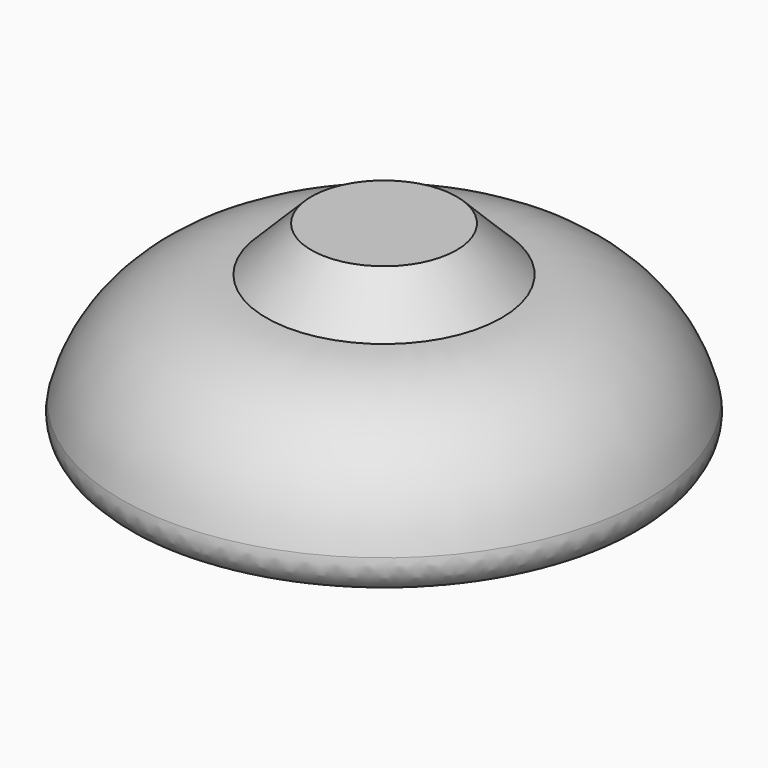
from build123d import *

# Parameters (mm, degrees)
F0_R     = 45.3065751062
F1_DEPTH = 25.4
F2_R     = 25.39999
F3_R     = 5.08
F4_T     = 2.54
F5_DEPTH = 7.62
F6_SIZE  = 7.61999
F7_DEPTH = 20.32
F8_R     = 19.812


# Not quite as in the source:
# - a fillet or chamfer is up to 0.001 mm smaller than in the source, because OpenCascade refuses the exact size
# - a shell that OpenCascade refuses in one call is made with other operations: the cavity is built on its own and cut out


with BuildPart() as f1:
    # F0 (on Top) → F1 (new body)
    with BuildSketch(Plane.XY):
        Circle(F0_R)
    extrude(amount=F1_DEPTH)

    # F2 (radius 25.4 in the source; OpenCascade refuses exactly that, so slightly less here)
    f2_edges = [f1.edges().sort_by_distance(p)[0] for p in [
        (-45.306575, 0, 25.4),
    ]]
    fillet(f2_edges, radius=F2_R)

    # F3
    f3_edges = [f1.edges().sort_by_distance(p)[0] for p in [
        (-45.306575, 0, 0),
    ]]
    fillet(f3_edges, radius=F3_R)

    # F4: shell of thickness 2.54, made by hand


with BuildPart() as f4_core1:
    # F4_t2: copy of F1
    add(f1.part)

    # the walls: a layer under each face that stays
    f4_faces = [f4_core1.faces().sort_by_distance(p)[0] for p in [
        (-35.4608426764, 0, 20.0804622717),
        (-43.5974247944, 0, 1.9691472612),
        (0, 0, 25.4),
    ]]
    thicken(f4_faces, amount=-F4_T, mode=Mode.SUBTRACT)


with BuildPart() as f1_1:
    add(f1.part)

    # what is left inside the walls is the cavity
    f4_cavity = [f4_core1.part.solids().sort_by_distance(p)[0] for p in [
        (-37.487808, 0, 14.571183),
    ]]
    add(f4_cavity, mode=Mode.SUBTRACT)

    # F5 (add): a face of the model
    f5_faces = [f1_1.faces().sort_by_distance(p)[0] for p in [
        (0, 0, 25.4),
    ]]
    extrude(f5_faces, amount=F5_DEPTH)

    # F6 (size 7.62 in the source; OpenCascade refuses exactly that, so slightly less here)
    f6_edges = [f1_1.edges().sort_by_distance(p)[0] for p in [
        (-19.906585, 0, 33.02),
    ]]
    chamfer(f6_edges, length=F6_SIZE)

    # F7 (add): a face of the model
    f7_faces = [f1_1.faces().sort_by_distance(p)[0] for p in [
        (-4.79e-08, 0, 22.86),
    ]]
    extrude(f7_faces, amount=F7_DEPTH)

    # F8
    f8_edges = [f1_1.edges().sort_by_distance(p)[0] for p in [
        (-19.906585, 0, 2.54),
    ]]
    fillet(f8_edges, radius=F8_R)


solid = f1_1.part
